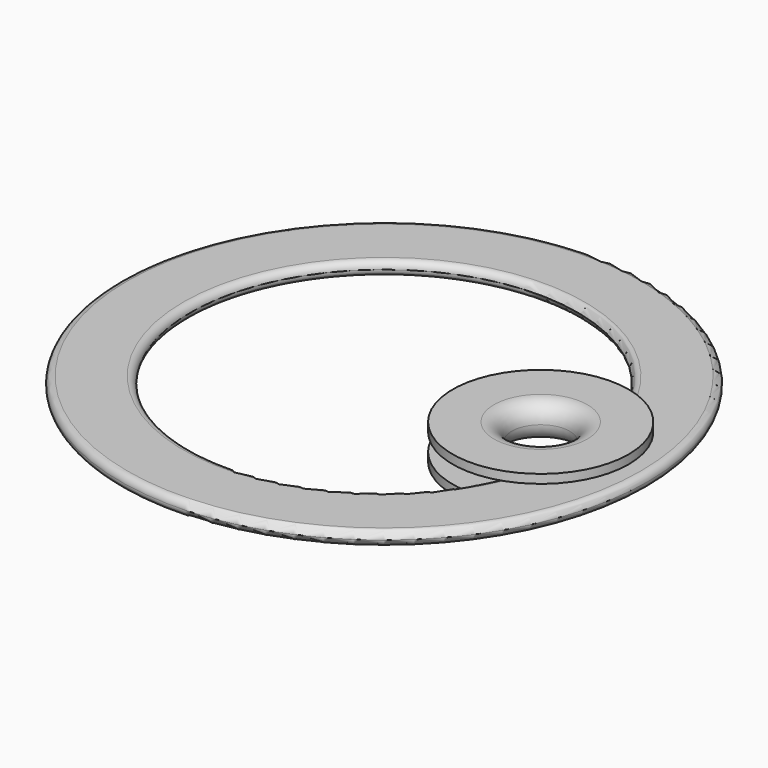
from build123d import *

# Parameters (mm, degrees)
F0_R     = 75
F0_R_2   = 55
F1_DEPTH = 4
F4_R     = 8.25
F5_DEPTH = 25
F6_R     = 4.99999
F7_R     = 1.99999
F7_2_R   = 1.99999
F8_R     = 1.99999


# Not quite as in the source:
# - a fillet or chamfer is up to 0.001 mm smaller than in the source, because OpenCascade refuses the exact size


with BuildPart() as f1:
    # F0 (on Top) → F1 (new body)
    with BuildSketch(Plane.XY):
        Circle(F0_R)
        Circle(F0_R_2, mode=Mode.SUBTRACT)
    extrude(amount=F1_DEPTH)

    # F7 (radius 2 in the source; OpenCascade refuses exactly that, so slightly less here)
    f7_edges = [f1.edges().sort_by_distance(p)[0] for p in [
        (55, 0, 2),
        (-55, 0, 0),
        (-55, 0, 4),
    ]]
    fillet(f7_edges, radius=F7_R)

    # F8 (radius 2 in the source; OpenCascade refuses exactly that, so slightly less here)
    f8_edges = [f1.edges().sort_by_distance(p)[0] for p in [
        (-75, 0, 4),
        (-75, 0, 0),
    ]]
    fillet(f8_edges, radius=F8_R)


with BuildPart() as f3:
    # F2 (on Front) → F3 (revolve)
    with BuildSketch(Plane.XZ):
        Polygon((54.5, -0.5), (54.5, 4.5), (69.5, 4.5), (69.5, 7), (54.5, 7), (44.5, 7), (44.5, -3), (54.5, -3), (69.5, -3), (69.5, -0.5), align=None)
    revolve(axis=Axis((44.5, 0, 2), (0, 0, 1)))

    # F4 (on face) → F5 (cut)
    with BuildSketch(Plane.XY.offset(7)):
        with Locations((44.5, 0)):
            Circle(F4_R)
    extrude(amount=-F5_DEPTH, mode=Mode.SUBTRACT)

    # F6 (radius 5 in the source; OpenCascade refuses exactly that, so slightly less here)
    f6_edges = [f3.edges().sort_by_distance(p)[0] for p in [
        (36.25, 0, 7),
        (36.25, 0, -3),
    ]]
    fillet(f6_edges, radius=F6_R)

    # F7#2 (radius 2 in the source; OpenCascade refuses exactly that, so slightly less here)
    f7_2_edges = [f3.edges().sort_by_distance(p)[0] for p in [
        (34.5, 0, -0.5),
        (34.5, 0, 4.5),
        (54.5, 0, 2),
    ]]
    fillet(f7_2_edges, radius=F7_2_R)


solid = Compound([f1.part, f3.part])
